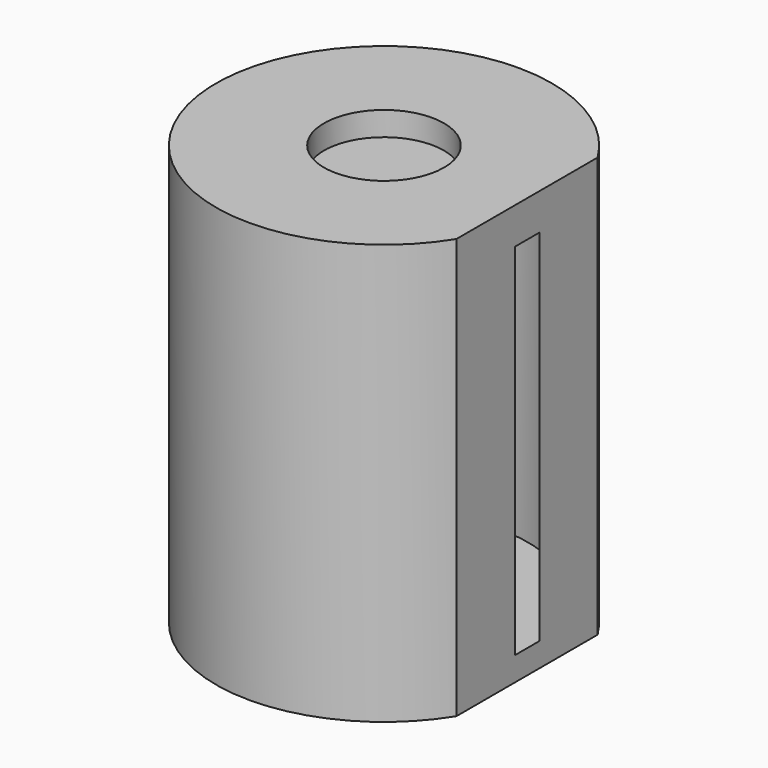
from build123d import *

# Parameters (mm, degrees)
F0_R      = 14
F2_DEPTH  = 35
F3_R      = 5
F4_DEPTH  = 5
F1_R      = 5
F5_DEPTH  = 5
F7_SCALE  = 0.856
F10_R     = 5
F10_R_2   = 4.28
F11_DEPTH = 3
F12_R     = 5
F12_R_2   = 4.28
F13_DEPTH = 3
F15_DEPTH = 41.7


with BuildPart() as f2:
    # F0 (on Top) → F2 (new body)
    with BuildSketch(Plane.XY):
        Circle(F0_R)
    extrude(amount=F2_DEPTH)

    # F3 (on face) → F4 (cut)
    with BuildSketch(Plane.XY.offset(35)):
        Circle(F3_R)
    extrude(amount=-F4_DEPTH, mode=Mode.SUBTRACT)

    # F1 (on Top) → F5 (cut)
    with BuildSketch(Plane.XY):
        Circle(F1_R)
    extrude(amount=F5_DEPTH, mode=Mode.SUBTRACT)


with BuildPart() as f6_1:
    # F6: copy of F2
    add(f2.part.moved(Location((0, 0, -2))))


with BuildPart() as f7_1:
    # F7: copy of F2
    add(f2.part.scale(F7_SCALE))


with BuildPart() as f6_1_1:
    add(f6_1.part)

    # F9: cut F7_1
    add(f7_1.part, mode=Mode.SUBTRACT)

    # F12 (on face) → F13 (join)
    with BuildSketch(Plane(origin=(0, 0, 3), x_dir=(1, 0, 0), z_dir=(0, 0, -1))):
        Circle(F12_R)
        Circle(F12_R_2, mode=Mode.SUBTRACT)
        Circle(F12_R_2)
    extrude(amount=F13_DEPTH)

    # F14 (on face) → F15 (cut)
    with BuildSketch(Plane.XY.offset(33)):
        with BuildLine():
            Line((11.9155967814, -7.349731515), (11.9155967814, -11.6381047294))
            Line((11.9155967814, -11.6381047294), (22.9155967814, -11.6381047294))
            Line((22.9155967814, -11.6381047294), (22.9155967814, 13.3618952706))
            Line((22.9155967814, 13.3618952706), (11.9155967814, 13.3618952706))
            Line((11.9155967814, 13.3618952706), (11.9155967814, 7.349731515))
            ThreePointArc((11.9155967814, 7.349731515), (13.4688224233, 3.8197935193), (14, 0))
            ThreePointArc((14, 0), (13.4688224233, -3.8197935193), (11.9155967814, -7.349731515))
        make_face()
        with BuildLine():
            Line((11.9155967814, 7.349731515), (11.9155967814, -7.349731515))
            ThreePointArc((11.9155967814, -7.349731515), (13.4688224233, -3.8197935193), (14, 0))
            ThreePointArc((14, 0), (13.4688224233, 3.8197935193), (11.9155967814, 7.349731515))
        make_face()
    extrude(amount=-F15_DEPTH, mode=Mode.SUBTRACT)


with BuildPart() as f11:
    # F10 (on face) → F11 (new body)
    with BuildSketch(Plane.XY.offset(28)):
        Circle(F10_R)
        Circle(F10_R_2, mode=Mode.SUBTRACT)
        Circle(F10_R_2)
    extrude(amount=F11_DEPTH)


solid = Compound([f6_1_1.part, f11.part])
